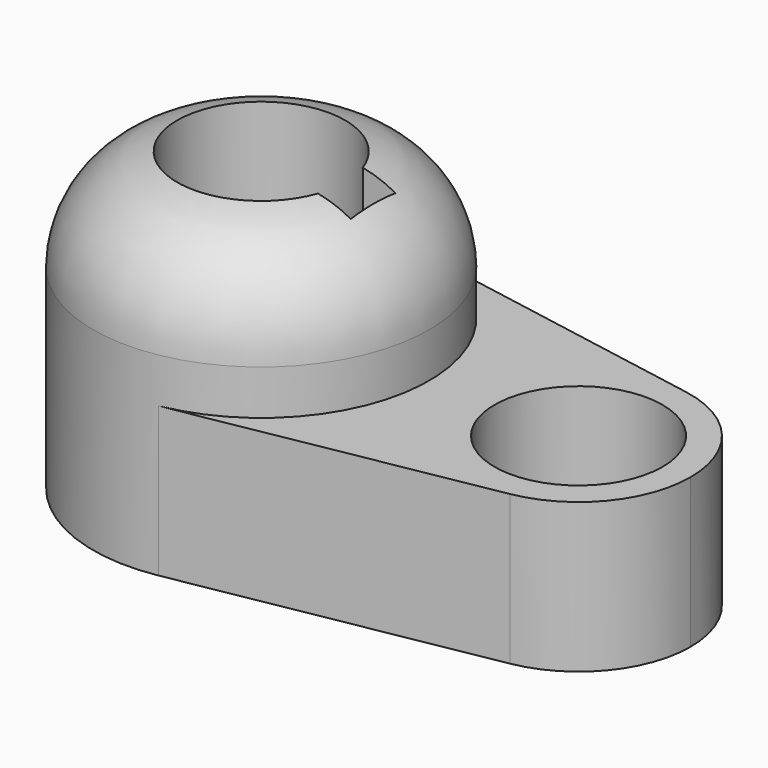
from build123d import *

# Parameters (mm, degrees)
F0_R     = 14.2875
F1_DEPTH = 25.4
F2_DEPTH = 50.8


# Not quite as in the source:
# - a fillet or chamfer that OpenCascade refuses, or shapes differently, is made with other operations: its cross-section is extruded or revolved along the edge and cut away or added


with BuildPart() as f1:
    # F0 (on Top) → F1 (new body)
    with BuildSketch(Plane.XY):
        with BuildLine():
            ThreePointArc((5.0426470588, -28.1265414802), (21.9160245563, -18.3362616868), (28.575, 0))
            ThreePointArc((28.575, 0), (21.9160245563, 18.3362616868), (5.0426470588, 28.1265414802))
            ThreePointArc((5.0426470588, 28.1265414802), (-28.575, 0), (5.0426470588, -28.1265414802))
        make_face()
        with BuildLine():
            ThreePointArc((-13.4703841816, 4.7625), (0, 14.2875), (13.4703841816, 4.7625))
            Line((13.4703841816, 4.7625), (19.05, 4.7625))
            Line((19.05, 4.7625), (19.05, -4.7625))
            Line((19.05, -4.7625), (13.4703841816, -4.7625))
            ThreePointArc((13.4703841816, -4.7625), (0, -14.2875), (-13.4703841816, -4.7625))
            Line((-13.4703841816, -4.7625), (-19.05, -4.7625))
            Line((-19.05, -4.7625), (-19.05, 4.7625))
            Line((-19.05, 4.7625), (-13.4703841816, 4.7625))
        make_face(mode=Mode.SUBTRACT)
        with BuildLine():
            ThreePointArc((5.0426470588, 28.1265414802), (21.9160245563, 18.3362616868), (28.575, 0))
            ThreePointArc((28.575, 0), (21.9160245563, -18.3362616868), (5.0426470588, -28.1265414802))
            Line((5.0426470588, -28.1265414802), (57.3367647059, -18.7510276535))
            ThreePointArc((57.3367647059, -18.7510276535), (34.925, 0), (57.3367647059, 18.7510276535))
            Line((57.3367647059, 18.7510276535), (5.0426470588, 28.1265414802))
        make_face()
        with BuildLine():
            ThreePointArc((-13.4703841816, -4.7625), (-14.2875, 0), (-13.4703841816, 4.7625))
            Line((-13.4703841816, 4.7625), (-19.05, 4.7625))
            Line((-19.05, 4.7625), (-19.05, -4.7625))
            Line((-19.05, -4.7625), (-13.4703841816, -4.7625))
        make_face()
        with BuildLine():
            ThreePointArc((73.025, 0), (68.5856830375, 12.2241744579), (57.3367647059, 18.7510276535))
            ThreePointArc((57.3367647059, 18.7510276535), (34.925, 0), (57.3367647059, -18.7510276535))
            ThreePointArc((57.3367647059, -18.7510276535), (68.5856830375, -12.2241744579), (73.025, 0))
        make_face()
        with Locations((53.975, 0)):
            Circle(F0_R, mode=Mode.SUBTRACT)
    extrude(amount=F1_DEPTH)

    # F0 (on Top) → F2 (join)
    with BuildSketch(Plane.XY):
        with BuildLine():
            ThreePointArc((5.0426470588, -28.1265414802), (21.9160245563, -18.3362616868), (28.575, 0))
            ThreePointArc((28.575, 0), (21.9160245563, 18.3362616868), (5.0426470588, 28.1265414802))
            ThreePointArc((5.0426470588, 28.1265414802), (-28.575, 0), (5.0426470588, -28.1265414802))
        make_face()
        with BuildLine():
            ThreePointArc((-13.4703841816, 4.7625), (0, 14.2875), (13.4703841816, 4.7625))
            Line((13.4703841816, 4.7625), (19.05, 4.7625))
            Line((19.05, 4.7625), (19.05, -4.7625))
            Line((19.05, -4.7625), (13.4703841816, -4.7625))
            ThreePointArc((13.4703841816, -4.7625), (0, -14.2875), (-13.4703841816, -4.7625))
            Line((-13.4703841816, -4.7625), (-19.05, -4.7625))
            Line((-19.05, -4.7625), (-19.05, 4.7625))
            Line((-19.05, 4.7625), (-13.4703841816, 4.7625))
        make_face(mode=Mode.SUBTRACT)
        with BuildLine():
            ThreePointArc((-13.4703841816, -4.7625), (-14.2875, 0), (-13.4703841816, 4.7625))
            Line((-13.4703841816, 4.7625), (-19.05, 4.7625))
            Line((-19.05, 4.7625), (-19.05, -4.7625))
            Line((-19.05, -4.7625), (-13.4703841816, -4.7625))
        make_face()
    extrude(amount=F2_DEPTH)

    # F3: fillet of radius 17.78 on 1 edges, made by hand

    # F3_s1 → F3_t2 (revolve, cut)
    with BuildSketch(Plane(origin=(0, 0, 0), x_dir=(0, 0, 1), z_dir=(-0.9843059136, -0.1764705882, 0))):
        with BuildLine():
            ThreePointArc((33.02, -28.575), (45.5923585695, -23.3673585695), (50.8, -10.795))
            Line((50.8, -10.795), (50.8, -28.575))
            Line((50.8, -28.575), (33.02, -28.575))
        make_face()
    revolve(axis=Axis((0, 0, 50.8), (0, 0, 1)), mode=Mode.SUBTRACT)


solid = f1.part
